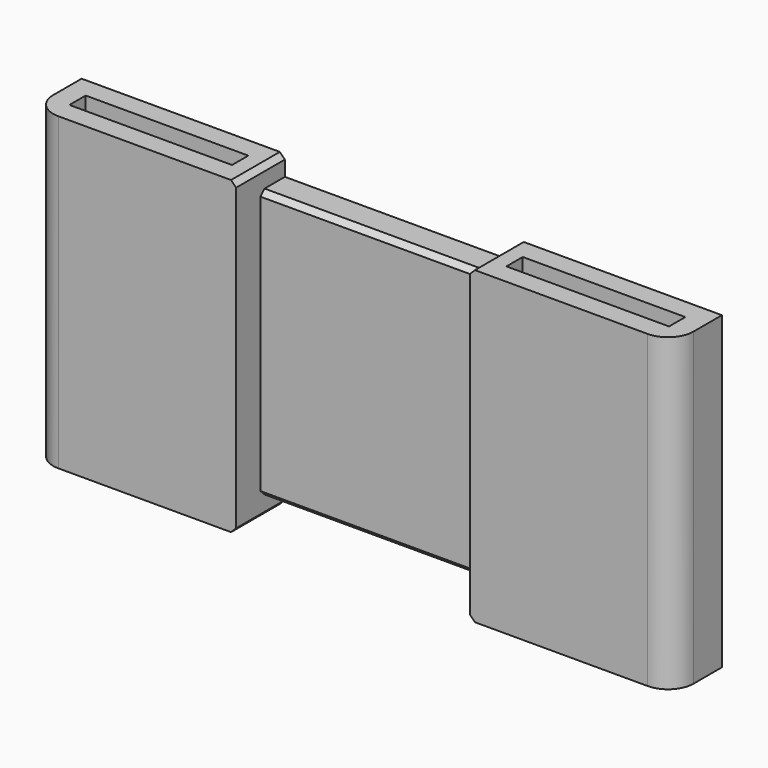
from build123d import *

# Parameters (mm, degrees)
F0_W     = 16
F0_H     = 2
F1_DEPTH = 30.5
F2_R     = 2.5
F3_W     = 23
F3_H     = 2
F4_DEPTH = 25
F5_SIZE  = 0.5


with BuildPart() as f1:
    # F0 (on Top) → F1 (new body)
    with BuildSketch(Plane.XY):
        Polygon((54.3318165131, 15.8888510838), (-8.6681834869, 15.8888510838), (-8.6681834869, 9.8888510838), (11.3318165131, 9.8888510838), (11.3318165131, 12.8888510838), (34.3318165131, 12.8888510838), (34.3318165131, 9.8888510838), (54.3318165131, 9.8888510838), align=None)
        with Locations((1.3318165131, 12.8888510838)):
            Rectangle(F0_W, F0_H, mode=Mode.SUBTRACT)
        with Locations((44.3318165131, 12.8888510838)):
            Rectangle(F0_W, F0_H, mode=Mode.SUBTRACT)
    extrude(amount=F1_DEPTH)

    # F2
    f2_edges = [f1.edges().sort_by_distance(p)[0] for p in [
        (-8.668183, 9.888851, 15.25),
        (54.331817, 9.888851, 15.25),
    ]]
    fillet(f2_edges, radius=F2_R)

    # F3 (on face) → F4 (cut)
    with BuildSketch(Plane.XZ.offset(-12.8888510838)):
        with Locations((22.8318165131, 1)):
            Rectangle(F3_W, F3_H)
        with Locations((22.8318165131, 29.5)):
            Rectangle(F3_W, F3_H)
    extrude(amount=-F4_DEPTH, mode=Mode.SUBTRACT)

    # F5
    f5_edges = [f1.edges().sort_by_distance(p)[0] for p in [
        (11.331817, 12.888851, 30.5),
        (34.331817, 12.888851, 30.5),
        (34.331817, 12.888851, 0),
        (11.331817, 12.888851, 0),
        (22.831817, 12.888851, 2),
        (22.831817, 12.888851, 28.5),
    ]]
    chamfer(f5_edges, length=F5_SIZE)


solid = f1.part
